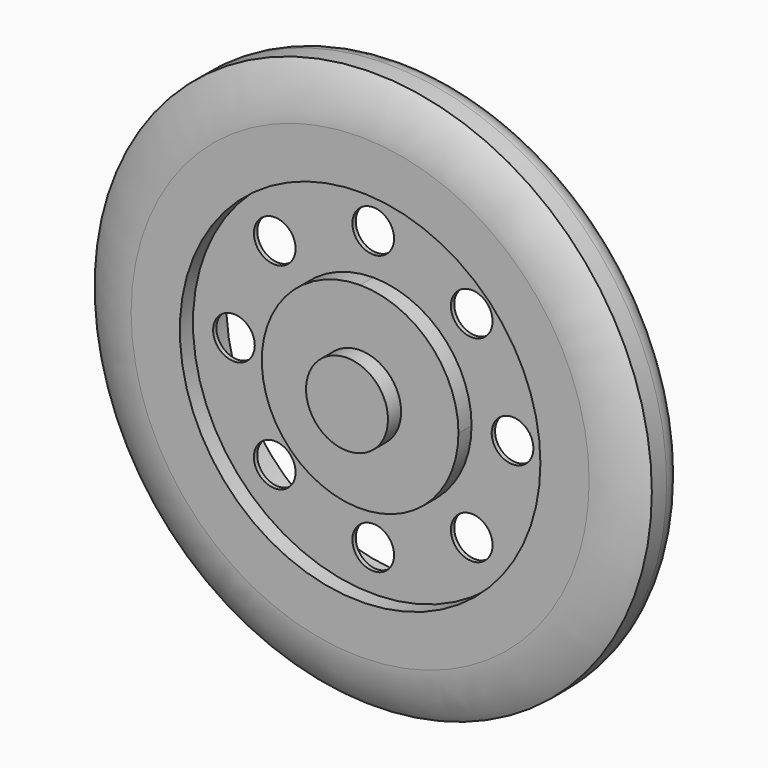
from build123d import *

# Parameters (mm, degrees)
F1_R     = 17
F1_R_2   = 11
F2_DEPTH = 1
F1_R_3   = 2.5
F3_DEPTH = 2
F1_R_4   = 1.2715293898
F4_DEPTH = 0.254
F6_DEPTH = 2.54
F7_R     = 1.4103835631


# Not quite as in the source:
# - a fillet or chamfer that OpenCascade refuses, or shapes differently, is made with other operations: its cross-section is extruded or revolved along the edge and cut away or added


with BuildPart() as f2:
    # F1 (on face) → F2 (new body)
    with BuildSketch(Plane.XZ):
        Circle(F1_R)
        Circle(F1_R_2, mode=Mode.SUBTRACT)
    extrude(amount=F2_DEPTH)

    # F5: fillet of radius 5.08 on 1 edges, made by hand

    # F5_s1 → F5_t2 (revolve, cut)
    with BuildSketch(Plane.XY):
        with BuildLine():
            ThreePointArc((17, 0), (15.567188555, -0.7435256815), (13.9734508099, -1))
            Line((13.9734508099, -1), (17, -1))
            Line((17, -1), (17, 0))
        make_face()
    revolve(axis=Axis((0, -1, 0), (0, -1, 0)), mode=Mode.SUBTRACT)


with BuildPart() as f2b:
    # F1 (on face) → F2, piece 2 (new body)
    with BuildSketch(Plane.XZ):
        with BuildLine():
            ThreePointArc((0, 6), (-4.2426406871, -4.2426406871), (6, 0))
            ThreePointArc((6, 0), (4.2426406871, 4.2426406871), (0, 6))
        make_face()
        Circle(F1_R_3, mode=Mode.SUBTRACT)
    extrude(amount=F2_DEPTH)

    # F1 (on face) → F3 (join)
    with BuildSketch(Plane.XZ):
        Circle(F1_R_3)
    extrude(amount=F3_DEPTH)


with BuildPart() as f4:
    # F1 (on face) → F4 (new body)
    with BuildSketch(Plane.XZ):
        Circle(F1_R_2)
        with Locations((-6.0104076401, -6.0104076401)):
            Circle(F1_R_4, mode=Mode.SUBTRACT)
        with Locations((0, -8.5)):
            Circle(F1_R_4, mode=Mode.SUBTRACT)
        with Locations((6.0104076401, -6.0104076401)):
            Circle(F1_R_4, mode=Mode.SUBTRACT)
        with Locations((-8.5, 0)):
            Circle(F1_R_4, mode=Mode.SUBTRACT)
        with Locations((-6.0104076401, 6.0104076401)):
            Circle(F1_R_4, mode=Mode.SUBTRACT)
        with BuildLine():
            ThreePointArc((0, 6), (4.2426406871, 4.2426406871), (6, 0))
            ThreePointArc((6, 0), (-4.2426406871, -4.2426406871), (0, 6))
        make_face(mode=Mode.SUBTRACT)
        with Locations((8.5, 0)):
            Circle(F1_R_4, mode=Mode.SUBTRACT)
        with BuildLine():
            ThreePointArc((1.2715293898, 8.5), (0.899107054, 7.600892946), (0, 7.2284706102))
            ThreePointArc((0, 7.2284706102), (-0.899107054, 9.399107054), (1.2715293898, 8.5))
        make_face(mode=Mode.SUBTRACT)
        with Locations((6.0104076401, 6.0104076401)):
            Circle(F1_R_4, mode=Mode.SUBTRACT)
    extrude(amount=-F4_DEPTH)


with BuildPart() as f6:
    # F1 (on face) → F6 (new body)
    with BuildSketch(Plane.XZ):
        Circle(F1_R)
        Circle(F1_R_2, mode=Mode.SUBTRACT)
    extrude(amount=-F6_DEPTH)

    # F7
    f7_edges = [f6.edges().sort_by_distance(p)[0] for p in [
        (-17, 2.54, 0),
    ]]
    fillet(f7_edges, radius=F7_R)


solid = Compound([f2.part, f2b.part, f4.part, f6.part])
